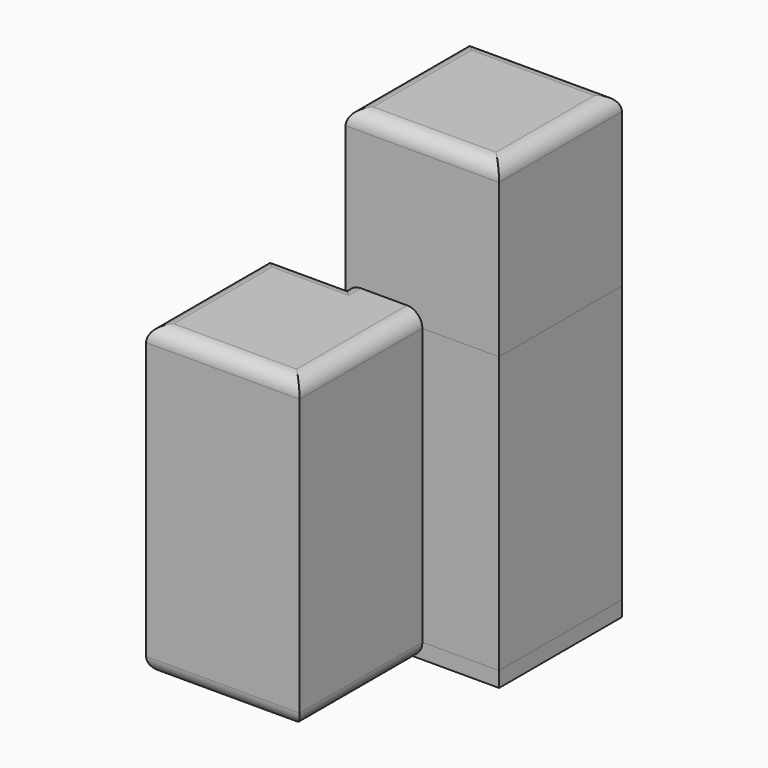
from build123d import *

# Parameters (mm, degrees)
F1_DEPTH       = 25.4
F3_DEPTH       = 76.2
F4_DEPTH       = 50.8
F5_R           = 2.7983271334
F6_DEPTH       = 40.64
F7_T1_DEPTH    = 38.1
F7_T3_DEPTH    = 38.1
F7_2_T1_DEPTH  = 31.75
F7_2_T3_DEPTH  = 19.05
F7_2_T5_DEPTH  = 38.1
F7_2_T7_DEPTH  = 38.1
F7_2_T9_DEPTH  = 31.75
F7_2_T11_DEPTH = 19.05
F7_2_T13_DEPTH = 38.1
F7_2_T15_DEPTH = 38.1
F7_2_T21_DEPTH = 38.1
F7_2_T25_DEPTH = 25.4
F7_2_T32_DEPTH = 38.1
F7_2_T36_DEPTH = 25.4
F7_2_T43_DEPTH = 38.1
F7_2_T47_DEPTH = 25.4
F7_2_T54_DEPTH = 38.1
F7_2_T58_DEPTH = 25.4
F7_3_T1_DEPTH  = 38.1
F7_3_T3_DEPTH  = 38.1


# Not quite as in the source:
# - a fillet or chamfer that OpenCascade refuses, or shapes differently, is made with other operations: its cross-section is extruded or revolved along the edge and cut away or added


with BuildPart() as f1:
    # F0 (on Top) → F1 (new body)
    with BuildSketch(Plane.XY):
        Polygon((-12.7, 0), (0, 0), (0, 25.4), (-25.4, 25.4), (-25.4, 0), align=None)
    extrude(amount=F1_DEPTH)

    # F5 (on face) → F6 (cut)
    with BuildSketch(Plane.XY.offset(25.4)):
        with Locations((-20.7387898117, 13.1304748356)):
            Circle(F5_R)
    extrude(amount=-F6_DEPTH, mode=Mode.SUBTRACT)

    # F7: fillet of radius 2.54 on 10 edges, made by hand

    # F7_s2 → F7_t1 (cut)
    with BuildSketch(Plane.YZ.offset(-31.75)):
        with BuildLine():
            ThreePointArc((0, 22.86), (0.7439487758, 24.6560512242), (2.54, 25.4))
            Line((2.54, 25.4), (0, 25.4))
            Line((0, 25.4), (0, 22.86))
        make_face()
        with BuildLine():
            ThreePointArc((22.86, 25.4), (24.6560512242, 24.6560512242), (25.4, 22.86))
            Line((25.4, 22.86), (25.4, 25.4))
            Line((25.4, 25.4), (22.86, 25.4))
        make_face()
        with BuildLine():
            ThreePointArc((0, 2.54), (0.7439487758, 0.7439487758), (2.54, 0))
            Line((2.54, 0), (0, 0))
            Line((0, 0), (0, 2.54))
        make_face()
        with BuildLine():
            ThreePointArc((22.86, 0), (24.6560512242, 0.7439487758), (25.4, 2.54))
            Line((25.4, 2.54), (25.4, 0))
            Line((25.4, 0), (22.86, 0))
        make_face()
    extrude(amount=F7_T1_DEPTH, mode=Mode.SUBTRACT)

    # F7_s4 → F7_t3 (cut)
    with BuildSketch(Plane.XZ.offset(-31.75)):
        with BuildLine():
            ThreePointArc((0, 22.86), (-0.7439487758, 24.6560512242), (-2.54, 25.4))
            Line((-2.54, 25.4), (0, 25.4))
            Line((0, 25.4), (0, 22.86))
        make_face()
        with BuildLine():
            ThreePointArc((-25.4, 22.86), (-24.6560512242, 24.6560512242), (-22.86, 25.4))
            Line((-22.86, 25.4), (-25.4, 25.4))
            Line((-25.4, 25.4), (-25.4, 22.86))
        make_face()
        with BuildLine():
            ThreePointArc((0, 2.54), (-0.7439487758, 0.7439487758), (-2.54, 0))
            Line((-2.54, 0), (0, 0))
            Line((0, 0), (0, 2.54))
        make_face()
        with BuildLine():
            ThreePointArc((-22.86, 0), (-24.6560512242, 0.7439487758), (-25.4, 2.54))
            Line((-25.4, 2.54), (-25.4, 0))
            Line((-25.4, 0), (-22.86, 0))
        make_face()
    extrude(amount=F7_T3_DEPTH, mode=Mode.SUBTRACT)

    # F7_s5 → F7_t6 (revolve, cut)
    with BuildSketch(Plane.XZ.offset(-13.1304748356)):
        with BuildLine():
            ThreePointArc((-15.4004626784, 25.4), (-17.1965139026, 24.6560512242), (-17.9404626784, 22.86))
            Line((-17.9404626784, 22.86), (-17.9404626784, 25.4))
            Line((-17.9404626784, 25.4), (-15.4004626784, 25.4))
        make_face()
    revolve(axis=Axis((-20.7387898117, 13.1304748356, 25.4), (0, 0, 1)), mode=Mode.SUBTRACT)

    # F7_s7 → F7_t8 (revolve, cut)
    with BuildSketch(Plane.XZ.offset(-13.1304748356)):
        with BuildLine():
            ThreePointArc((-15.4004626784, 0), (-17.1965139026, 0.7439487758), (-17.9404626784, 2.54))
            Line((-17.9404626784, 2.54), (-17.9404626784, 0))
            Line((-17.9404626784, 0), (-15.4004626784, 0))
        make_face()
    revolve(axis=Axis((-20.7387898117, 13.1304748356, 0), (0, 0, 1)), mode=Mode.SUBTRACT)


with BuildPart() as f3:
    # F2 (on Top) → F3 (new body)
    with BuildSketch(Plane.XY):
        Polygon((0, 25.4), (0, 0), (12.7, 0), (25.4, 0), (25.4, 25.4), align=None)
    extrude(amount=F3_DEPTH)

    # F7#3: fillet of radius 2.54 on 4 edges, made by hand

    # F7_3_s2 → F7_3_t1 (cut)
    with BuildSketch(Plane.XZ.offset(-31.75)):
        with BuildLine():
            ThreePointArc((0, 73.66), (0.7439487758, 75.4560512242), (2.54, 76.2))
            Line((2.54, 76.2), (0, 76.2))
            Line((0, 76.2), (0, 73.66))
        make_face()
        with BuildLine():
            ThreePointArc((22.86, 76.2), (24.6560512242, 75.4560512242), (25.4, 73.66))
            Line((25.4, 73.66), (25.4, 76.2))
            Line((25.4, 76.2), (22.86, 76.2))
        make_face()
    extrude(amount=F7_3_T1_DEPTH, mode=Mode.SUBTRACT)

    # F7_3_s4 → F7_3_t3 (cut)
    with BuildSketch(Plane.YZ.offset(-6.35)):
        with BuildLine():
            ThreePointArc((2.54, 76.2), (0.7439487758, 75.4560512242), (0, 73.66))
            Line((0, 73.66), (0, 76.2))
            Line((0, 76.2), (2.54, 76.2))
        make_face()
        with BuildLine():
            ThreePointArc((22.86, 76.2), (24.6560512242, 75.4560512242), (25.4, 73.66))
            Line((25.4, 73.66), (25.4, 76.2))
            Line((25.4, 76.2), (22.86, 76.2))
        make_face()
    extrude(amount=F7_3_T3_DEPTH, mode=Mode.SUBTRACT)


with BuildPart() as f4:
    # F2 (on Top) → F4 (new body)
    with BuildSketch(Plane.XY):
        Polygon((0, 25.4), (0, 0), (12.7, 0), (25.4, 0), (25.4, 25.4), align=None)
        Polygon((12.7, 0), (0, 0), (-12.7, 0), (-12.7, -25.4), (12.7, -25.4), align=None)
    extrude(amount=F4_DEPTH)

    # F7#2: fillet of radius 2.54 on 16 edges, made by hand

    # F7_2_s2 → F7_2_t1 (cut)
    with BuildSketch(Plane.XZ.offset(-31.75)):
        with BuildLine():
            ThreePointArc((0, 2.54), (0.7439487758, 0.7439487758), (2.54, 0))
            Line((2.54, 0), (0, 0))
            Line((0, 0), (0, 2.54))
        make_face()
        with BuildLine():
            ThreePointArc((0, 48.26), (0.7439487758, 50.0560512242), (2.54, 50.8))
            Line((2.54, 50.8), (0, 50.8))
            Line((0, 50.8), (0, 48.26))
        make_face()
    extrude(amount=F7_2_T1_DEPTH, mode=Mode.SUBTRACT)

    # F7_2_s4 → F7_2_t3 (cut)
    with BuildSketch(Plane.YZ.offset(-19.05)):
        with BuildLine():
            ThreePointArc((0, 48.26), (-0.7439487758, 50.0560512242), (-2.54, 50.8))
            Line((-2.54, 50.8), (0, 50.8))
            Line((0, 50.8), (0, 48.26))
        make_face()
        with BuildLine():
            ThreePointArc((0, 2.54), (-0.7439487758, 0.7439487758), (-2.54, 0))
            Line((-2.54, 0), (0, 0))
            Line((0, 0), (0, 2.54))
        make_face()
    extrude(amount=F7_2_T3_DEPTH, mode=Mode.SUBTRACT)

    # F7_2_s6 → F7_2_t5 (cut)
    with BuildSketch(Plane.XZ.offset(-6.35)):
        with BuildLine():
            ThreePointArc((-12.7, 48.26), (-11.9560512242, 50.0560512242), (-10.16, 50.8))
            Line((-10.16, 50.8), (-12.7, 50.8))
            Line((-12.7, 50.8), (-12.7, 48.26))
        make_face()
        with BuildLine():
            ThreePointArc((-12.7, 2.54), (-11.9560512242, 0.7439487758), (-10.16, 0))
            Line((-10.16, 0), (-12.7, 0))
            Line((-12.7, 0), (-12.7, 2.54))
        make_face()
    extrude(amount=F7_2_T5_DEPTH, mode=Mode.SUBTRACT)

    # F7_2_s8 → F7_2_t7 (cut)
    with BuildSketch(Plane.YZ.offset(-19.05)):
        with BuildLine():
            ThreePointArc((-25.4, 48.26), (-24.6560512242, 50.0560512242), (-22.86, 50.8))
            Line((-22.86, 50.8), (-25.4, 50.8))
            Line((-25.4, 50.8), (-25.4, 48.26))
        make_face()
        with BuildLine():
            ThreePointArc((-25.4, 2.54), (-24.6560512242, 0.7439487758), (-22.86, 0))
            Line((-22.86, 0), (-25.4, 0))
            Line((-25.4, 0), (-25.4, 2.54))
        make_face()
    extrude(amount=F7_2_T7_DEPTH, mode=Mode.SUBTRACT)

    # F7_2_s10 → F7_2_t9 (cut)
    with BuildSketch(Plane.XZ):
        with BuildLine():
            ThreePointArc((12.7, 48.26), (11.9560512242, 50.0560512242), (10.16, 50.8))
            Line((10.16, 50.8), (12.7, 50.8))
            Line((12.7, 50.8), (12.7, 48.26))
        make_face()
        with BuildLine():
            ThreePointArc((12.7, 2.54), (11.9560512242, 0.7439487758), (10.16, 0))
            Line((10.16, 0), (12.7, 0))
            Line((12.7, 0), (12.7, 2.54))
        make_face()
    extrude(amount=F7_2_T9_DEPTH, mode=Mode.SUBTRACT)

    # F7_2_s12 → F7_2_t11 (cut)
    with BuildSketch(Plane.YZ.offset(12.7)):
        with BuildLine():
            ThreePointArc((0, 48.26), (0.7439487758, 50.0560512242), (2.54, 50.8))
            Line((2.54, 50.8), (0, 50.8))
            Line((0, 50.8), (0, 48.26))
        make_face()
        with BuildLine():
            ThreePointArc((0, 2.54), (0.7439487758, 0.7439487758), (2.54, 0))
            Line((2.54, 0), (0, 0))
            Line((0, 0), (0, 2.54))
        make_face()
    extrude(amount=F7_2_T11_DEPTH, mode=Mode.SUBTRACT)

    # F7_2_s14 → F7_2_t13 (cut)
    with BuildSketch(Plane.XZ.offset(-31.75)):
        with BuildLine():
            ThreePointArc((25.4, 48.26), (24.6560512242, 50.0560512242), (22.86, 50.8))
            Line((22.86, 50.8), (25.4, 50.8))
            Line((25.4, 50.8), (25.4, 48.26))
        make_face()
        with BuildLine():
            ThreePointArc((25.4, 2.54), (24.6560512242, 0.7439487758), (22.86, 0))
            Line((22.86, 0), (25.4, 0))
            Line((25.4, 0), (25.4, 2.54))
        make_face()
    extrude(amount=F7_2_T13_DEPTH, mode=Mode.SUBTRACT)

    # F7_2_s16 → F7_2_t15 (cut)
    with BuildSketch(Plane.YZ.offset(-6.35)):
        with BuildLine():
            ThreePointArc((25.4, 48.26), (24.6560512242, 50.0560512242), (22.86, 50.8))
            Line((22.86, 50.8), (25.4, 50.8))
            Line((25.4, 50.8), (25.4, 48.26))
        make_face()
        with BuildLine():
            ThreePointArc((25.4, 2.54), (24.6560512242, 0.7439487758), (22.86, 0))
            Line((22.86, 0), (25.4, 0))
            Line((25.4, 0), (25.4, 2.54))
        make_face()
    extrude(amount=F7_2_T15_DEPTH, mode=Mode.SUBTRACT)


with BuildPart() as f7_2_tool19:
    # F7_2_s20 → F7_2_t21 (new body)
    with BuildSketch(Plane.XZ.offset(-31.75)):
        with BuildLine():
            ThreePointArc((0, 2.54), (0.7439487758, 0.7439487758), (2.54, 0))
            Line((2.54, 0), (0, 0))
            Line((0, 0), (0, 2.54))
        make_face()
    extrude(amount=F7_2_T21_DEPTH)

    split(bisect_by=Plane.XZ, keep=Keep.TOP)


with BuildPart() as f7_2_tool23:
    # F7_2_s24 → F7_2_t25 (new body)
    with BuildSketch(Plane.YZ.offset(6.35)):
        with BuildLine():
            ThreePointArc((0, 2.54), (-0.7439487758, 0.7439487758), (-2.54, 0))
            Line((-2.54, 0), (0, 0))
            Line((0, 0), (0, 2.54))
        make_face()
    extrude(amount=-F7_2_T25_DEPTH)

    split(bisect_by=Plane.YZ, keep=Keep.TOP)


with BuildPart() as f7_2_tool19_1:
    add(f7_2_tool19.part)

    # F7_2_t27: intersect F7_2_tool23
    add(f7_2_tool23.part, mode=Mode.INTERSECT)


with BuildPart() as f4_1:
    add(f4.part)

    # F7_2_t17: cut F7_2_tool19
    add(f7_2_tool19_1.part, mode=Mode.SUBTRACT)


with BuildPart() as f7_2_tool30:
    # F7_2_s31 → F7_2_t32 (new body)
    with BuildSketch(Plane.XZ.offset(-31.75)):
        with BuildLine():
            ThreePointArc((0, 48.26), (0.7439487758, 50.0560512242), (2.54, 50.8))
            Line((2.54, 50.8), (0, 50.8))
            Line((0, 50.8), (0, 48.26))
        make_face()
    extrude(amount=F7_2_T32_DEPTH)

    split(bisect_by=Plane.XZ, keep=Keep.TOP)


with BuildPart() as f7_2_tool34:
    # F7_2_s35 → F7_2_t36 (new body)
    with BuildSketch(Plane.YZ.offset(6.35)):
        with BuildLine():
            ThreePointArc((0, 48.26), (-0.7439487758, 50.0560512242), (-2.54, 50.8))
            Line((-2.54, 50.8), (0, 50.8))
            Line((0, 50.8), (0, 48.26))
        make_face()
    extrude(amount=-F7_2_T36_DEPTH)

    split(bisect_by=Plane.YZ, keep=Keep.TOP)


with BuildPart() as f7_2_tool30_1:
    add(f7_2_tool30.part)

    # F7_2_t38: intersect F7_2_tool34
    add(f7_2_tool34.part, mode=Mode.INTERSECT)


with BuildPart() as f4_2:
    add(f4_1.part)

    # F7_2_t28: cut F7_2_tool30
    add(f7_2_tool30_1.part, mode=Mode.SUBTRACT)


with BuildPart() as f7_2_tool41:
    # F7_2_s42 → F7_2_t43 (new body)
    with BuildSketch(Plane.XZ.offset(31.75)):
        with BuildLine():
            ThreePointArc((12.7, 48.26), (11.9560512242, 50.0560512242), (10.16, 50.8))
            Line((10.16, 50.8), (12.7, 50.8))
            Line((12.7, 50.8), (12.7, 48.26))
        make_face()
    extrude(amount=-F7_2_T43_DEPTH)

    split(bisect_by=Plane.XZ, keep=Keep.BOTTOM)


with BuildPart() as f7_2_tool45:
    # F7_2_s46 → F7_2_t47 (new body)
    with BuildSketch(Plane.YZ.offset(6.35)):
        with BuildLine():
            ThreePointArc((0, 48.26), (0.7439487758, 50.0560512242), (2.54, 50.8))
            Line((2.54, 50.8), (0, 50.8))
            Line((0, 50.8), (0, 48.26))
        make_face()
    extrude(amount=F7_2_T47_DEPTH)

    split(bisect_by=Plane.YZ.offset(12.7), keep=Keep.BOTTOM)


with BuildPart() as f7_2_tool41_1:
    add(f7_2_tool41.part)

    # F7_2_t49: intersect F7_2_tool45
    add(f7_2_tool45.part, mode=Mode.INTERSECT)


with BuildPart() as f4_3:
    add(f4_2.part)

    # F7_2_t39: cut F7_2_tool41
    add(f7_2_tool41_1.part, mode=Mode.SUBTRACT)


with BuildPart() as f7_2_tool52:
    # F7_2_s53 → F7_2_t54 (new body)
    with BuildSketch(Plane.XZ.offset(31.75)):
        with BuildLine():
            ThreePointArc((12.7, 2.54), (11.9560512242, 0.7439487758), (10.16, 0))
            Line((10.16, 0), (12.7, 0))
            Line((12.7, 0), (12.7, 2.54))
        make_face()
    extrude(amount=-F7_2_T54_DEPTH)

    split(bisect_by=Plane.XZ, keep=Keep.BOTTOM)


with BuildPart() as f7_2_tool56:
    # F7_2_s57 → F7_2_t58 (new body)
    with BuildSketch(Plane.YZ.offset(6.35)):
        with BuildLine():
            ThreePointArc((0, 2.54), (0.7439487758, 0.7439487758), (2.54, 0))
            Line((2.54, 0), (0, 0))
            Line((0, 0), (0, 2.54))
        make_face()
    extrude(amount=F7_2_T58_DEPTH)

    split(bisect_by=Plane.YZ.offset(12.7), keep=Keep.BOTTOM)


with BuildPart() as f7_2_tool52_1:
    add(f7_2_tool52.part)

    # F7_2_t60: intersect F7_2_tool56
    add(f7_2_tool56.part, mode=Mode.INTERSECT)


with BuildPart() as f4_4:
    add(f4_3.part)

    # F7_2_t50: cut F7_2_tool52
    add(f7_2_tool52_1.part, mode=Mode.SUBTRACT)


solid = Compound([f1.part, f3.part, f4_4.part])
